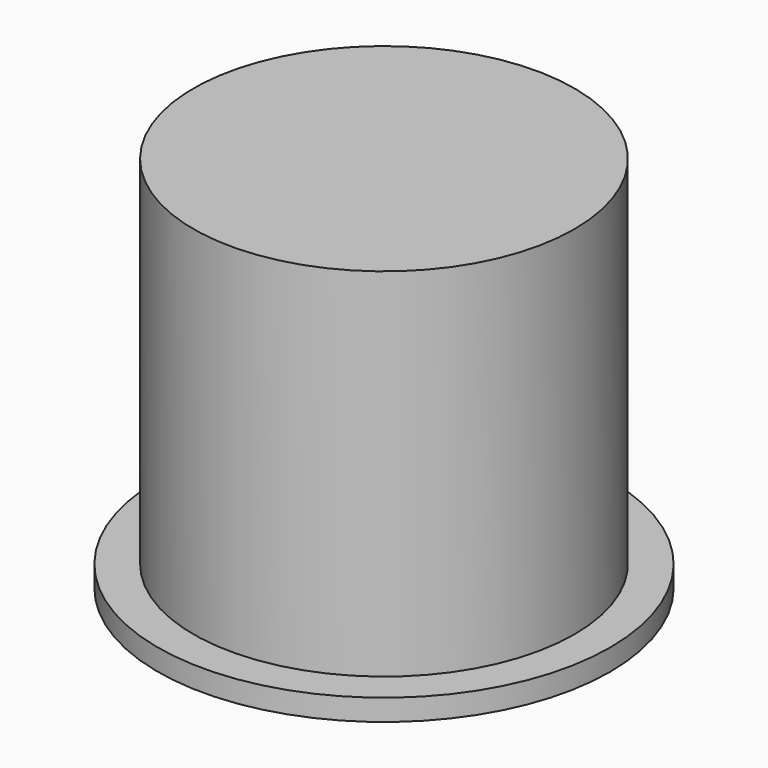
from build123d import *

# Parameters (mm, degrees)
F0_R     = 26.7
F0_R_2   = 24.7
F1_DEPTH = 50
F2_R     = 26.7
F3_DEPTH = 3
F4_R     = 31.7
F4_R_2   = 26.7
F4_R_3   = 24.7
F5_DEPTH = 3


with BuildPart() as f1:
    # F0 (on Top) → F1 (new body)
    with BuildSketch(Plane.XY):
        Circle(F0_R)
        Circle(F0_R_2, mode=Mode.SUBTRACT)
    extrude(amount=F1_DEPTH)

    # F2 (on face) → F3 (join)
    with BuildSketch(Plane.XY.offset(50)):
        Circle(F2_R)
    extrude(amount=F3_DEPTH)

    # F4 (on face) → F5 (join)
    with BuildSketch(Plane(origin=(0, 0, 0), x_dir=(1, 0, 0), z_dir=(0, 0, -1))):
        Circle(F4_R)
        Circle(F4_R_2, mode=Mode.SUBTRACT)
        Circle(F4_R_2)
        Circle(F4_R_3, mode=Mode.SUBTRACT)
    extrude(amount=-F5_DEPTH)


solid = f1.part
